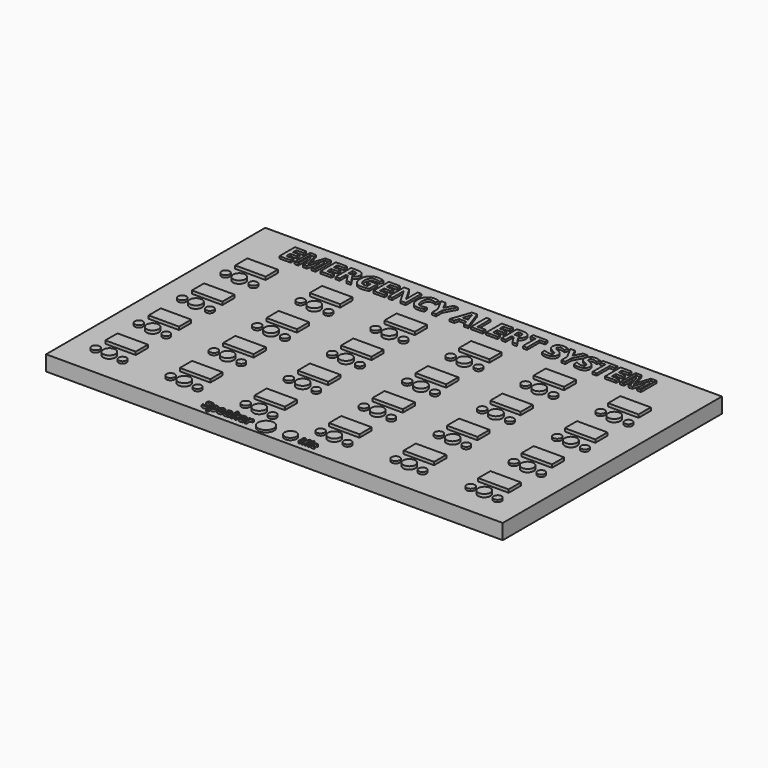
from build123d import *

# Parameters (mm, degrees)
F0_W          = 1500
F0_H          = 900
F1_DEPTH      = 50
F2_W          = 100
F2_H          = 50
F3_DEPTH      = 10
F4_R          = 20.1444297478
F5_DEPTH      = 10
F7_R          = 12.7
F8_DEPTH      = 7
F9_R          = 13.5588842663
F10_DEPTH     = 7
F11_TEXT_SIZE = 89.4236481852
F12_DEPTH     = 7
F13_R         = 26.0019215875
F14_DEPTH     = 7
F15_R         = 19.2698910709
F16_DEPTH     = 7
F17_TEXT_SIZE = 38.9928619067
F18_DEPTH     = 7
F19_TEXT_SIZE = 31.1942978038
F20_DEPTH     = 7
F21_DEPTH     = 7
F22_DEPTH     = 7


# Not quite as in the source:
# - Text() gives the source's letters only with a copy of the font that has no kerning and outlines rounded to 1/6400 em; it was checked with that copy


with BuildPart() as f1:
    # F0 (on Top) → F1 (new body)
    with BuildSketch(Plane.XY):
        Rectangle(F0_W, F0_H)
    extrude(amount=F1_DEPTH)


with BuildPart() as f3:
    # F2 (on face) → F3 (new body)
    with BuildSketch(Plane.XY.offset(50)):
        with Locations((-617.6470518112, 248.6287260949)):
            Rectangle(F2_W, F2_H)
    extrude(amount=F3_DEPTH)


with BuildPart() as f3b:
    # F2 (on face) → F3, piece 2 (new body)
    with BuildSketch(Plane.XY.offset(50)):
        with Locations((-617.6470518112, 70.8287260949)):
            Rectangle(F2_W, F2_H)
    extrude(amount=F3_DEPTH)


with BuildPart() as f3c:
    # F2 (on face) → F3, piece 3 (new body)
    with BuildSketch(Plane.XY.offset(50)):
        with Locations((-617.6470518112, -106.9712739051)):
            Rectangle(F2_W, F2_H)
    extrude(amount=F3_DEPTH)


with BuildPart() as f3d:
    # F2 (on face) → F3, piece 4 (new body)
    with BuildSketch(Plane.XY.offset(50)):
        with Locations((-617.6470518112, -284.7712739051)):
            Rectangle(F2_W, F2_H)
    extrude(amount=F3_DEPTH)


with BuildPart() as f3e:
    # F2 (on face) → F3, piece 5 (new body)
    with BuildSketch(Plane.XY.offset(50)):
        with Locations((-372.6470518112, 248.6287260949)):
            Rectangle(F2_W, F2_H)
    extrude(amount=F3_DEPTH)


with BuildPart() as f3f:
    # F2 (on face) → F3, piece 6 (new body)
    with BuildSketch(Plane.XY.offset(50)):
        with Locations((-372.6470518112, 70.8287260949)):
            Rectangle(F2_W, F2_H)
    extrude(amount=F3_DEPTH)


with BuildPart() as f3g:
    # F2 (on face) → F3, piece 7 (new body)
    with BuildSketch(Plane.XY.offset(50)):
        with Locations((-372.6470518112, -106.9712739051)):
            Rectangle(F2_W, F2_H)
    extrude(amount=F3_DEPTH)


with BuildPart() as f3h:
    # F2 (on face) → F3, piece 8 (new body)
    with BuildSketch(Plane.XY.offset(50)):
        with Locations((-372.6470518112, -284.7712739051)):
            Rectangle(F2_W, F2_H)
    extrude(amount=F3_DEPTH)


with BuildPart() as f3i:
    # F2 (on face) → F3, piece 9 (new body)
    with BuildSketch(Plane.XY.offset(50)):
        with Locations((-127.6470518112, 248.6287260949)):
            Rectangle(F2_W, F2_H)
    extrude(amount=F3_DEPTH)


with BuildPart() as f3j:
    # F2 (on face) → F3, piece 10 (new body)
    with BuildSketch(Plane.XY.offset(50)):
        with Locations((-127.6470518112, 70.8287260949)):
            Rectangle(F2_W, F2_H)
    extrude(amount=F3_DEPTH)


with BuildPart() as f3k:
    # F2 (on face) → F3, piece 11 (new body)
    with BuildSketch(Plane.XY.offset(50)):
        with Locations((-127.6470518112, -106.9712739051)):
            Rectangle(F2_W, F2_H)
    extrude(amount=F3_DEPTH)


with BuildPart() as f3l:
    # F2 (on face) → F3, piece 12 (new body)
    with BuildSketch(Plane.XY.offset(50)):
        with Locations((-127.6470518112, -284.7712739051)):
            Rectangle(F2_W, F2_H)
    extrude(amount=F3_DEPTH)


with BuildPart() as f3m:
    # F2 (on face) → F3, piece 13 (new body)
    with BuildSketch(Plane.XY.offset(50)):
        with Locations((117.3529481888, 248.6287260949)):
            Rectangle(F2_W, F2_H)
    extrude(amount=F3_DEPTH)


with BuildPart() as f3n:
    # F2 (on face) → F3, piece 14 (new body)
    with BuildSketch(Plane.XY.offset(50)):
        with Locations((117.3529481888, 70.8287260949)):
            Rectangle(F2_W, F2_H)
    extrude(amount=F3_DEPTH)


with BuildPart() as f3o:
    # F2 (on face) → F3, piece 15 (new body)
    with BuildSketch(Plane.XY.offset(50)):
        with Locations((117.3529481888, -106.9712739051)):
            Rectangle(F2_W, F2_H)
    extrude(amount=F3_DEPTH)


with BuildPart() as f3p:
    # F2 (on face) → F3, piece 16 (new body)
    with BuildSketch(Plane.XY.offset(50)):
        with Locations((117.3529481888, -284.7712739051)):
            Rectangle(F2_W, F2_H)
    extrude(amount=F3_DEPTH)


with BuildPart() as f3q:
    # F2 (on face) → F3, piece 17 (new body)
    with BuildSketch(Plane.XY.offset(50)):
        with Locations((362.3529481888, 248.6287260949)):
            Rectangle(F2_W, F2_H)
    extrude(amount=F3_DEPTH)


with BuildPart() as f3r:
    # F2 (on face) → F3, piece 18 (new body)
    with BuildSketch(Plane.XY.offset(50)):
        with Locations((362.3529481888, 70.8287260949)):
            Rectangle(F2_W, F2_H)
    extrude(amount=F3_DEPTH)


with BuildPart() as f3s:
    # F2 (on face) → F3, piece 19 (new body)
    with BuildSketch(Plane.XY.offset(50)):
        with Locations((362.3529481888, -106.9712739051)):
            Rectangle(F2_W, F2_H)
    extrude(amount=F3_DEPTH)


with BuildPart() as f3t:
    # F2 (on face) → F3, piece 20 (new body)
    with BuildSketch(Plane.XY.offset(50)):
        with Locations((362.3529481888, -284.7712739051)):
            Rectangle(F2_W, F2_H)
    extrude(amount=F3_DEPTH)


with BuildPart() as f3u:
    # F2 (on face) → F3, piece 21 (new body)
    with BuildSketch(Plane.XY.offset(50)):
        with Locations((607.3529481888, 248.6287260949)):
            Rectangle(F2_W, F2_H)
    extrude(amount=F3_DEPTH)


with BuildPart() as f3v:
    # F2 (on face) → F3, piece 22 (new body)
    with BuildSketch(Plane.XY.offset(50)):
        with Locations((607.3529481888, 70.8287260949)):
            Rectangle(F2_W, F2_H)
    extrude(amount=F3_DEPTH)


with BuildPart() as f3w:
    # F2 (on face) → F3, piece 23 (new body)
    with BuildSketch(Plane.XY.offset(50)):
        with Locations((607.3529481888, -106.9712739051)):
            Rectangle(F2_W, F2_H)
    extrude(amount=F3_DEPTH)


with BuildPart() as f3x:
    # F2 (on face) → F3, piece 24 (new body)
    with BuildSketch(Plane.XY.offset(50)):
        with Locations((607.3529481888, -284.7712739051)):
            Rectangle(F2_W, F2_H)
    extrude(amount=F3_DEPTH)


with BuildPart() as f5:
    # F4 (on face) → F5 (new body)
    with BuildSketch(Plane.XY.offset(50)):
        with Locations((-619.8930740356, 180.4278045893)):
            Circle(F4_R)
    extrude(amount=F5_DEPTH)


with BuildPart() as f5b:
    # F4 (on face) → F5, piece 2 (new body)
    with BuildSketch(Plane.XY.offset(50)):
        with Locations((-619.8930740356, 2.6278045893)):
            Circle(F4_R)
    extrude(amount=F5_DEPTH)


with BuildPart() as f5c:
    # F4 (on face) → F5, piece 3 (new body)
    with BuildSketch(Plane.XY.offset(50)):
        with Locations((-619.8930740356, -175.1721954107)):
            Circle(F4_R)
    extrude(amount=F5_DEPTH)


with BuildPart() as f5d:
    # F4 (on face) → F5, piece 4 (new body)
    with BuildSketch(Plane.XY.offset(50)):
        with Locations((-619.8930740356, -352.9721954107)):
            Circle(F4_R)
    extrude(amount=F5_DEPTH)


with BuildPart() as f5e:
    # F4 (on face) → F5, piece 5 (new body)
    with BuildSketch(Plane.XY.offset(50)):
        with Locations((-373.5130740356, 180.4278045893)):
            Circle(F4_R)
    extrude(amount=F5_DEPTH)


with BuildPart() as f5f:
    # F4 (on face) → F5, piece 6 (new body)
    with BuildSketch(Plane.XY.offset(50)):
        with Locations((-373.5130740356, 2.6278045893)):
            Circle(F4_R)
    extrude(amount=F5_DEPTH)


with BuildPart() as f5g:
    # F4 (on face) → F5, piece 7 (new body)
    with BuildSketch(Plane.XY.offset(50)):
        with Locations((-373.5130740356, -175.1721954107)):
            Circle(F4_R)
    extrude(amount=F5_DEPTH)


with BuildPart() as f5h:
    # F4 (on face) → F5, piece 8 (new body)
    with BuildSketch(Plane.XY.offset(50)):
        with Locations((-373.5130740356, -352.9721954107)):
            Circle(F4_R)
    extrude(amount=F5_DEPTH)


with BuildPart() as f5i:
    # F4 (on face) → F5, piece 9 (new body)
    with BuildSketch(Plane.XY.offset(50)):
        with Locations((-127.1330740356, 180.4278045893)):
            Circle(F4_R)
    extrude(amount=F5_DEPTH)


with BuildPart() as f5j:
    # F4 (on face) → F5, piece 10 (new body)
    with BuildSketch(Plane.XY.offset(50)):
        with Locations((-127.1330740356, 2.6278045893)):
            Circle(F4_R)
    extrude(amount=F5_DEPTH)


with BuildPart() as f5k:
    # F4 (on face) → F5, piece 11 (new body)
    with BuildSketch(Plane.XY.offset(50)):
        with Locations((-127.1330740356, -175.1721954107)):
            Circle(F4_R)
    extrude(amount=F5_DEPTH)


with BuildPart() as f5l:
    # F4 (on face) → F5, piece 12 (new body)
    with BuildSketch(Plane.XY.offset(50)):
        with Locations((-127.1330740356, -352.9721954107)):
            Circle(F4_R)
    extrude(amount=F5_DEPTH)


with BuildPart() as f5m:
    # F4 (on face) → F5, piece 13 (new body)
    with BuildSketch(Plane.XY.offset(50)):
        with Locations((119.2469259644, 180.4278045893)):
            Circle(F4_R)
    extrude(amount=F5_DEPTH)


with BuildPart() as f5n:
    # F4 (on face) → F5, piece 14 (new body)
    with BuildSketch(Plane.XY.offset(50)):
        with Locations((119.2469259644, 2.6278045893)):
            Circle(F4_R)
    extrude(amount=F5_DEPTH)


with BuildPart() as f5o:
    # F4 (on face) → F5, piece 15 (new body)
    with BuildSketch(Plane.XY.offset(50)):
        with Locations((119.2469259644, -175.1721954107)):
            Circle(F4_R)
    extrude(amount=F5_DEPTH)


with BuildPart() as f5p:
    # F4 (on face) → F5, piece 16 (new body)
    with BuildSketch(Plane.XY.offset(50)):
        with Locations((119.2469259644, -352.9721954107)):
            Circle(F4_R)
    extrude(amount=F5_DEPTH)


with BuildPart() as f5q:
    # F4 (on face) → F5, piece 17 (new body)
    with BuildSketch(Plane.XY.offset(50)):
        with Locations((365.6269259644, 180.4278045893)):
            Circle(F4_R)
    extrude(amount=F5_DEPTH)


with BuildPart() as f5r:
    # F4 (on face) → F5, piece 18 (new body)
    with BuildSketch(Plane.XY.offset(50)):
        with Locations((365.6269259644, 2.6278045893)):
            Circle(F4_R)
    extrude(amount=F5_DEPTH)


with BuildPart() as f5s:
    # F4 (on face) → F5, piece 19 (new body)
    with BuildSketch(Plane.XY.offset(50)):
        with Locations((365.6269259644, -175.1721954107)):
            Circle(F4_R)
    extrude(amount=F5_DEPTH)


with BuildPart() as f5t:
    # F4 (on face) → F5, piece 20 (new body)
    with BuildSketch(Plane.XY.offset(50)):
        with Locations((365.6269259644, -352.9721954107)):
            Circle(F4_R)
    extrude(amount=F5_DEPTH)


with BuildPart() as f5u:
    # F4 (on face) → F5, piece 21 (new body)
    with BuildSketch(Plane.XY.offset(50)):
        with Locations((612.0069259644, 180.4278045893)):
            Circle(F4_R)
    extrude(amount=F5_DEPTH)


with BuildPart() as f5v:
    # F4 (on face) → F5, piece 22 (new body)
    with BuildSketch(Plane.XY.offset(50)):
        with Locations((612.0069259644, 2.6278045893)):
            Circle(F4_R)
    extrude(amount=F5_DEPTH)


with BuildPart() as f5w:
    # F4 (on face) → F5, piece 23 (new body)
    with BuildSketch(Plane.XY.offset(50)):
        with Locations((612.0069259644, -175.1721954107)):
            Circle(F4_R)
    extrude(amount=F5_DEPTH)


with BuildPart() as f5x:
    # F4 (on face) → F5, piece 24 (new body)
    with BuildSketch(Plane.XY.offset(50)):
        with Locations((612.0069259644, -352.9721954107)):
            Circle(F4_R)
    extrude(amount=F5_DEPTH)


with BuildPart() as f8:
    # F7 (on face) → F8 (new body)
    with BuildSketch(Plane.XY.offset(50)):
        with Locations((-571.9786286354, 178.9304763079)):
            Circle(F7_R)
    extrude(amount=F8_DEPTH)


with BuildPart() as f8b:
    # F7 (on face) → F8, piece 2 (new body)
    with BuildSketch(Plane.XY.offset(50)):
        with Locations((-571.9786286354, -0.1395236921)):
            Circle(F7_R)
    extrude(amount=F8_DEPTH)


with BuildPart() as f8c:
    # F7 (on face) → F8, piece 3 (new body)
    with BuildSketch(Plane.XY.offset(50)):
        with Locations((-571.9786286354, -179.2095236921)):
            Circle(F7_R)
    extrude(amount=F8_DEPTH)


with BuildPart() as f8d:
    # F7 (on face) → F8, piece 4 (new body)
    with BuildSketch(Plane.XY.offset(50)):
        with Locations((-571.9786286354, -358.2795236921)):
            Circle(F7_R)
    extrude(amount=F8_DEPTH)


with BuildPart() as f8e:
    # F7 (on face) → F8, piece 5 (new body)
    with BuildSketch(Plane.XY.offset(50)):
        with Locations((-325.5986286354, 178.9304763079)):
            Circle(F7_R)
    extrude(amount=F8_DEPTH)


with BuildPart() as f8f:
    # F7 (on face) → F8, piece 6 (new body)
    with BuildSketch(Plane.XY.offset(50)):
        with Locations((-325.5986286354, -0.1395236921)):
            Circle(F7_R)
    extrude(amount=F8_DEPTH)


with BuildPart() as f8g:
    # F7 (on face) → F8, piece 7 (new body)
    with BuildSketch(Plane.XY.offset(50)):
        with Locations((-325.5986286354, -179.2095236921)):
            Circle(F7_R)
    extrude(amount=F8_DEPTH)


with BuildPart() as f8h:
    # F7 (on face) → F8, piece 8 (new body)
    with BuildSketch(Plane.XY.offset(50)):
        with Locations((-325.5986286354, -358.2795236921)):
            Circle(F7_R)
    extrude(amount=F8_DEPTH)


with BuildPart() as f8i:
    # F7 (on face) → F8, piece 9 (new body)
    with BuildSketch(Plane.XY.offset(50)):
        with Locations((-79.2186286354, 178.9304763079)):
            Circle(F7_R)
    extrude(amount=F8_DEPTH)


with BuildPart() as f8j:
    # F7 (on face) → F8, piece 10 (new body)
    with BuildSketch(Plane.XY.offset(50)):
        with Locations((-79.2186286354, -0.1395236921)):
            Circle(F7_R)
    extrude(amount=F8_DEPTH)


with BuildPart() as f8k:
    # F7 (on face) → F8, piece 11 (new body)
    with BuildSketch(Plane.XY.offset(50)):
        with Locations((-79.2186286354, -179.2095236921)):
            Circle(F7_R)
    extrude(amount=F8_DEPTH)


with BuildPart() as f8l:
    # F7 (on face) → F8, piece 12 (new body)
    with BuildSketch(Plane.XY.offset(50)):
        with Locations((-79.2186286354, -358.2795236921)):
            Circle(F7_R)
    extrude(amount=F8_DEPTH)


with BuildPart() as f8m:
    # F7 (on face) → F8, piece 13 (new body)
    with BuildSketch(Plane.XY.offset(50)):
        with Locations((167.1613713646, 178.9304763079)):
            Circle(F7_R)
    extrude(amount=F8_DEPTH)


with BuildPart() as f8n:
    # F7 (on face) → F8, piece 14 (new body)
    with BuildSketch(Plane.XY.offset(50)):
        with Locations((167.1613713646, -0.1395236921)):
            Circle(F7_R)
    extrude(amount=F8_DEPTH)


with BuildPart() as f8o:
    # F7 (on face) → F8, piece 15 (new body)
    with BuildSketch(Plane.XY.offset(50)):
        with Locations((167.1613713646, -179.2095236921)):
            Circle(F7_R)
    extrude(amount=F8_DEPTH)


with BuildPart() as f8p:
    # F7 (on face) → F8, piece 16 (new body)
    with BuildSketch(Plane.XY.offset(50)):
        with Locations((167.1613713646, -358.2795236921)):
            Circle(F7_R)
    extrude(amount=F8_DEPTH)


with BuildPart() as f8q:
    # F7 (on face) → F8, piece 17 (new body)
    with BuildSketch(Plane.XY.offset(50)):
        with Locations((413.5413713646, 178.9304763079)):
            Circle(F7_R)
    extrude(amount=F8_DEPTH)


with BuildPart() as f8r:
    # F7 (on face) → F8, piece 18 (new body)
    with BuildSketch(Plane.XY.offset(50)):
        with Locations((413.5413713646, -0.1395236921)):
            Circle(F7_R)
    extrude(amount=F8_DEPTH)


with BuildPart() as f8s:
    # F7 (on face) → F8, piece 19 (new body)
    with BuildSketch(Plane.XY.offset(50)):
        with Locations((413.5413713646, -179.2095236921)):
            Circle(F7_R)
    extrude(amount=F8_DEPTH)


with BuildPart() as f8t:
    # F7 (on face) → F8, piece 20 (new body)
    with BuildSketch(Plane.XY.offset(50)):
        with Locations((413.5413713646, -358.2795236921)):
            Circle(F7_R)
    extrude(amount=F8_DEPTH)


with BuildPart() as f8u:
    # F7 (on face) → F8, piece 21 (new body)
    with BuildSketch(Plane.XY.offset(50)):
        with Locations((659.9213713646, 178.9304763079)):
            Circle(F7_R)
    extrude(amount=F8_DEPTH)


with BuildPart() as f8v:
    # F7 (on face) → F8, piece 22 (new body)
    with BuildSketch(Plane.XY.offset(50)):
        with Locations((659.9213713646, -0.1395236921)):
            Circle(F7_R)
    extrude(amount=F8_DEPTH)


with BuildPart() as f8w:
    # F7 (on face) → F8, piece 23 (new body)
    with BuildSketch(Plane.XY.offset(50)):
        with Locations((659.9213713646, -179.2095236921)):
            Circle(F7_R)
    extrude(amount=F8_DEPTH)


with BuildPart() as f8x:
    # F7 (on face) → F8, piece 24 (new body)
    with BuildSketch(Plane.XY.offset(50)):
        with Locations((659.9213713646, -358.2795236921)):
            Circle(F7_R)
    extrude(amount=F8_DEPTH)


with BuildPart() as f10:
    # F9 (on face) → F10 (new body)
    with BuildSketch(Plane.XY.offset(50)):
        with Locations((-664.8128628731, 180.4278045893)):
            Circle(F9_R)
    extrude(amount=F10_DEPTH)


with BuildPart() as f10b:
    # F9 (on face) → F10, piece 2 (new body)
    with BuildSketch(Plane.XY.offset(50)):
        with Locations((-664.8128628731, 2.6278045893)):
            Circle(F9_R)
    extrude(amount=F10_DEPTH)


with BuildPart() as f10c:
    # F9 (on face) → F10, piece 3 (new body)
    with BuildSketch(Plane.XY.offset(50)):
        with Locations((-664.8128628731, -175.1721954107)):
            Circle(F9_R)
    extrude(amount=F10_DEPTH)


with BuildPart() as f10d:
    # F9 (on face) → F10, piece 4 (new body)
    with BuildSketch(Plane.XY.offset(50)):
        with Locations((-664.8128628731, -352.9721954107)):
            Circle(F9_R)
    extrude(amount=F10_DEPTH)


with BuildPart() as f10e:
    # F9 (on face) → F10, piece 5 (new body)
    with BuildSketch(Plane.XY.offset(50)):
        with Locations((-418.4328628731, 180.4278045893)):
            Circle(F9_R)
    extrude(amount=F10_DEPTH)


with BuildPart() as f10f:
    # F9 (on face) → F10, piece 6 (new body)
    with BuildSketch(Plane.XY.offset(50)):
        with Locations((-418.4328628731, 2.6278045893)):
            Circle(F9_R)
    extrude(amount=F10_DEPTH)


with BuildPart() as f10g:
    # F9 (on face) → F10, piece 7 (new body)
    with BuildSketch(Plane.XY.offset(50)):
        with Locations((-418.4328628731, -175.1721954107)):
            Circle(F9_R)
    extrude(amount=F10_DEPTH)


with BuildPart() as f10h:
    # F9 (on face) → F10, piece 8 (new body)
    with BuildSketch(Plane.XY.offset(50)):
        with Locations((-418.4328628731, -352.9721954107)):
            Circle(F9_R)
    extrude(amount=F10_DEPTH)


with BuildPart() as f10i:
    # F9 (on face) → F10, piece 9 (new body)
    with BuildSketch(Plane.XY.offset(50)):
        with Locations((-172.0528628731, 180.4278045893)):
            Circle(F9_R)
    extrude(amount=F10_DEPTH)


with BuildPart() as f10j:
    # F9 (on face) → F10, piece 10 (new body)
    with BuildSketch(Plane.XY.offset(50)):
        with Locations((-172.0528628731, 2.6278045893)):
            Circle(F9_R)
    extrude(amount=F10_DEPTH)


with BuildPart() as f10k:
    # F9 (on face) → F10, piece 11 (new body)
    with BuildSketch(Plane.XY.offset(50)):
        with Locations((-172.0528628731, -175.1721954107)):
            Circle(F9_R)
    extrude(amount=F10_DEPTH)


with BuildPart() as f10l:
    # F9 (on face) → F10, piece 12 (new body)
    with BuildSketch(Plane.XY.offset(50)):
        with Locations((-172.0528628731, -352.9721954107)):
            Circle(F9_R)
    extrude(amount=F10_DEPTH)


with BuildPart() as f10m:
    # F9 (on face) → F10, piece 13 (new body)
    with BuildSketch(Plane.XY.offset(50)):
        with Locations((74.3271371269, 180.4278045893)):
            Circle(F9_R)
    extrude(amount=F10_DEPTH)


with BuildPart() as f10n:
    # F9 (on face) → F10, piece 14 (new body)
    with BuildSketch(Plane.XY.offset(50)):
        with Locations((74.3271371269, 2.6278045893)):
            Circle(F9_R)
    extrude(amount=F10_DEPTH)


with BuildPart() as f10o:
    # F9 (on face) → F10, piece 15 (new body)
    with BuildSketch(Plane.XY.offset(50)):
        with Locations((74.3271371269, -175.1721954107)):
            Circle(F9_R)
    extrude(amount=F10_DEPTH)


with BuildPart() as f10p:
    # F9 (on face) → F10, piece 16 (new body)
    with BuildSketch(Plane.XY.offset(50)):
        with Locations((74.3271371269, -352.9721954107)):
            Circle(F9_R)
    extrude(amount=F10_DEPTH)


with BuildPart() as f10q:
    # F9 (on face) → F10, piece 17 (new body)
    with BuildSketch(Plane.XY.offset(50)):
        with Locations((320.7071371269, 180.4278045893)):
            Circle(F9_R)
    extrude(amount=F10_DEPTH)


with BuildPart() as f10r:
    # F9 (on face) → F10, piece 18 (new body)
    with BuildSketch(Plane.XY.offset(50)):
        with Locations((320.7071371269, 2.6278045893)):
            Circle(F9_R)
    extrude(amount=F10_DEPTH)


with BuildPart() as f10s:
    # F9 (on face) → F10, piece 19 (new body)
    with BuildSketch(Plane.XY.offset(50)):
        with Locations((320.7071371269, -175.1721954107)):
            Circle(F9_R)
    extrude(amount=F10_DEPTH)


with BuildPart() as f10t:
    # F9 (on face) → F10, piece 20 (new body)
    with BuildSketch(Plane.XY.offset(50)):
        with Locations((320.7071371269, -352.9721954107)):
            Circle(F9_R)
    extrude(amount=F10_DEPTH)


with BuildPart() as f10u:
    # F9 (on face) → F10, piece 21 (new body)
    with BuildSketch(Plane.XY.offset(50)):
        with Locations((567.0871371269, 180.4278045893)):
            Circle(F9_R)
    extrude(amount=F10_DEPTH)


with BuildPart() as f10v:
    # F9 (on face) → F10, piece 22 (new body)
    with BuildSketch(Plane.XY.offset(50)):
        with Locations((567.0871371269, 2.6278045893)):
            Circle(F9_R)
    extrude(amount=F10_DEPTH)


with BuildPart() as f10w:
    # F9 (on face) → F10, piece 23 (new body)
    with BuildSketch(Plane.XY.offset(50)):
        with Locations((567.0871371269, -175.1721954107)):
            Circle(F9_R)
    extrude(amount=F10_DEPTH)


with BuildPart() as f10x:
    # F9 (on face) → F10, piece 24 (new body)
    with BuildSketch(Plane.XY.offset(50)):
        with Locations((567.0871371269, -352.9721954107)):
            Circle(F9_R)
    extrude(amount=F10_DEPTH)


with BuildPart() as f12:
    # F11 (on face) → F12 (new body)
    with BuildSketch(Plane.XY.offset(50)):
        with Locations((-622.8877305984, 339.1443789005)):
            Text('EMERGENCY ALERT SYSTEM', F11_TEXT_SIZE, font='Open Sans', font_style=FontStyle.BOLD, text_align=(TextAlign.LEFT, TextAlign.BOTTOM))
    extrude(amount=F12_DEPTH)


with BuildPart() as f14:
    # F13 (on face) → F14 (new body)
    with BuildSketch(Plane.XY.offset(50)):
        with Locations((-54.2780794203, -416.4438247681)):
            Circle(F13_R)
    extrude(amount=F14_DEPTH)


with BuildPart() as f16:
    # F15 (on face) → F16 (new body)
    with BuildSketch(Plane.XY.offset(50)):
        with Locations((26.203205809, -416.4438247681)):
            Circle(F15_R)
    extrude(amount=F16_DEPTH)


with BuildPart() as f18:
    # F17 (on face) → F18 (new body)
    with BuildSketch(Plane.XY.offset(50)):
        with Locations((-256.4171105623, -431.4171373844)):
            Text('Speaker', F17_TEXT_SIZE, font='Open Sans', font_style=FontStyle.BOLD, text_align=(TextAlign.LEFT, TextAlign.BOTTOM))
    extrude(amount=F18_DEPTH)


with BuildPart() as f20:
    # F19 (on face) → F20 (new body)
    with BuildSketch(Plane.XY.offset(50)):
        with Locations((61.7647133768, -431.4171075821)):
            Text('Mic', F19_TEXT_SIZE, font='Open Sans', font_style=FontStyle.BOLD, text_align=(TextAlign.LEFT, TextAlign.BOTTOM))
    extrude(amount=F20_DEPTH)


with BuildPart() as f21:
    # F17 (on face) → F21 (new body)
    with BuildSketch(Plane.XY.offset(50)):
        with Locations((-256.4171105623, -431.4171373844)):
            Text('Speaker', F17_TEXT_SIZE, font='Open Sans', font_style=FontStyle.BOLD, text_align=(TextAlign.LEFT, TextAlign.BOTTOM))
    extrude(amount=F21_DEPTH)


with BuildPart() as f22:
    # F17 (on face) → F22 (new body)
    with BuildSketch(Plane.XY.offset(50)):
        with Locations((-256.4171105623, -431.4171373844)):
            Text('Speaker', F17_TEXT_SIZE, font='Open Sans', font_style=FontStyle.BOLD, text_align=(TextAlign.LEFT, TextAlign.BOTTOM))
    extrude(amount=F22_DEPTH)


solid = Compound([f1.part, f3.part, f3b.part, f3c.part, f3d.part, f3e.part, f3f.part, f3g.part, f3h.part, f3i.part, f3j.part, f3k.part, f3l.part, f3m.part, f3n.part, f3o.part, f3p.part, f3q.part, f3r.part, f3s.part, f3t.part, f3u.part, f3v.part, f3w.part, f3x.part, f5.part, f5b.part, f5c.part, f5d.part, f5e.part, f5f.part, f5g.part, f5h.part, f5i.part, f5j.part, f5k.part, f5l.part, f5m.part, f5n.part, f5o.part, f5p.part, f5q.part, f5r.part, f5s.part, f5t.part, f5u.part, f5v.part, f5w.part, f5x.part, f8.part, f8b.part, f8c.part, f8d.part, f8e.part, f8f.part, f8g.part, f8h.part, f8i.part, f8j.part, f8k.part, f8l.part, f8m.part, f8n.part, f8o.part, f8p.part, f8q.part, f8r.part, f8s.part, f8t.part, f8u.part, f8v.part, f8w.part, f8x.part, f10.part, f10b.part, f10c.part, f10d.part, f10e.part, f10f.part, f10g.part, f10h.part, f10i.part, f10j.part, f10k.part, f10l.part, f10m.part, f10n.part, f10o.part, f10p.part, f10q.part, f10r.part, f10s.part, f10t.part, f10u.part, f10v.part, f10w.part, f10x.part, f12.part, f14.part, f16.part, f18.part, f20.part, f21.part, f22.part])
